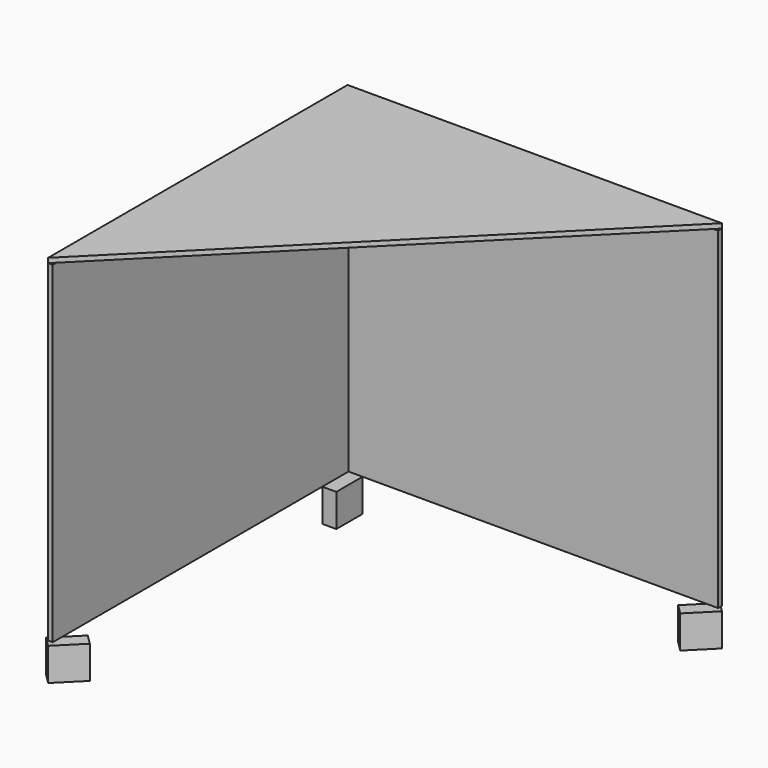
from build123d import *

# Parameters (mm, degrees)
F2_W      = 1016
F2_H      = 901.7
F3_DEPTH  = 12.7
F4_W      = 1016
F4_H      = 901.7
F5_DEPTH  = 12.7
F6_W      = 88.9
F6_H      = 88.9
F7_DEPTH  = 38.1
F8_W      = 38.1
F8_H      = 88.9
F9_DEPTH  = 88.9
F11_DEPTH = 12.7


with BuildPart() as f3:
    # F2 (on face) → F3 (new body)
    with BuildSketch(Plane(origin=(0, 453.2457475339, 0), x_dir=(-1, 0, 0), z_dir=(0, 1, 0))):
        with Locations((508, 463.55)):
            Rectangle(F2_W, F2_H)
    extrude(amount=-F3_DEPTH)

    # F4 (on face) → F5 (join)
    with BuildSketch(Plane(origin=(-1016, 0, 0), x_dir=(0, -1, 0), z_dir=(-1, 0, 0))):
        with Locations((54.7542524661, 463.55)):
            Rectangle(F4_W, F4_H)
    extrude(amount=-F5_DEPTH)

    # F10 (on face) → F11 (join)
    with BuildSketch(Plane.XY.offset(914.4)):
        Polygon((-1016, 453.2457475339), (-1016, -562.7542524661), (0, 453.2457475339), align=None)
    extrude(amount=F11_DEPTH)


with BuildPart() as f7:
    # F6 (on face) → F7 (new body)
    with BuildSketch(Plane(origin=(-226.6228737669, 226.6228737669, 0), x_dir=(0.7071067812, 0.7071067812, 0), z_dir=(0.7071067812, -0.7071067812, 0))):
        with Locations((-1071.8978377459, -44.45)):
            Rectangle(F6_W, F6_H)
    extrude(amount=-F7_DEPTH)


with BuildPart() as f7b:
    # F6 (on face) → F7, piece 2 (new body)
    with BuildSketch(Plane(origin=(-226.6228737669, 226.6228737669, 0), x_dir=(0.7071067812, 0.7071067812, 0), z_dir=(0.7071067812, -0.7071067812, 0))):
        with Locations((276.0431416252, -44.45)):
            Rectangle(F6_W, F6_H)
    extrude(amount=-F7_DEPTH)


with BuildPart() as f9:
    # F8 (on face) → F9 (new body)
    with BuildSketch(Plane(origin=(0, 0, 12.7), x_dir=(1, 0, 0), z_dir=(0, 0, -1))):
        with Locations((-984.25, -396.0957475339)):
            Rectangle(F8_W, F8_H)
    extrude(amount=F9_DEPTH)


solid = Compound([f3.part, f7.part, f7b.part, f9.part])
